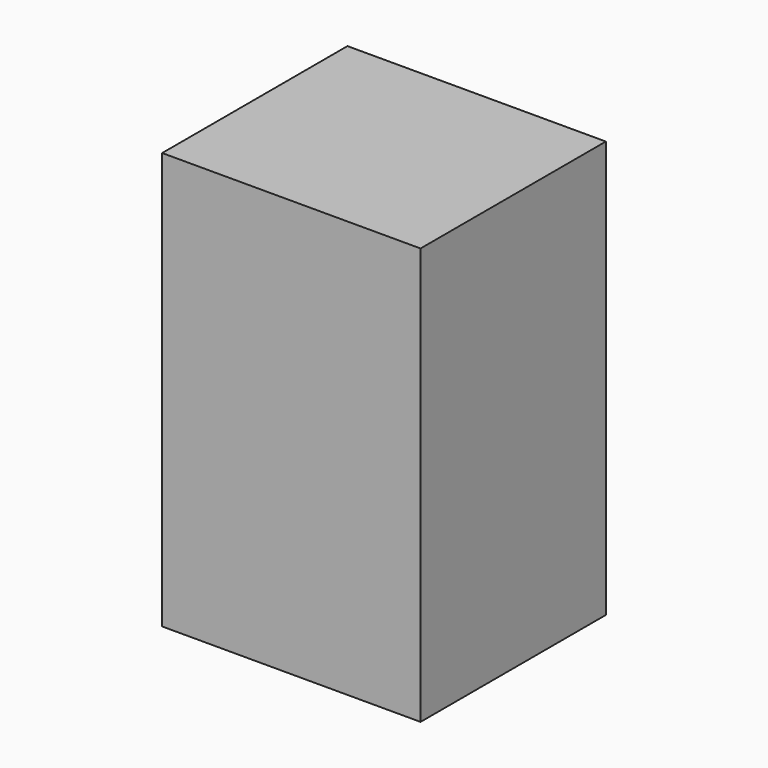
from build123d import *

# Parameters (mm, degrees)
F0_W     = 61.9848258793
F0_H     = 55.5620715022
F1_DEPTH = 100


# Not quite as in the source:
# - the program builds the solid bodies; features that only make, move or delete a surface that nothing else refers to are left out


with BuildPart() as f1:
    # F0 (on Top) → F1 (new body)
    with BuildSketch(Plane.XY):
        Rectangle(F0_W, F0_H)
    extrude(amount=F1_DEPTH)


solid = f1.part
